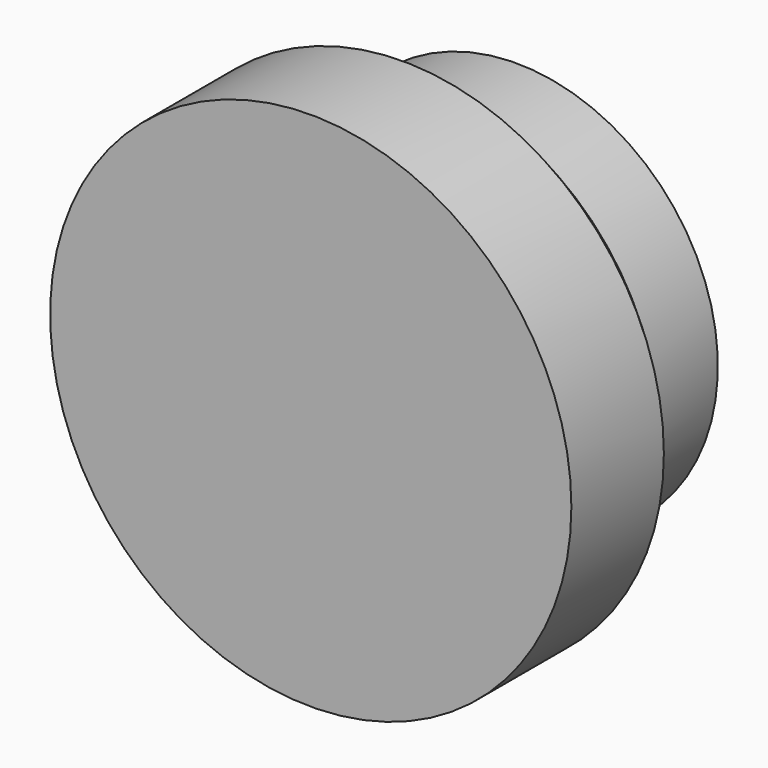
from build123d import *

# Parameters (mm, degrees)
F0_R     = 45.9871931788
F1_DEPTH = 12.7
F4_R     = 35.5142998493
F5_DEPTH = 20
F6_SIZE  = 5


# Not quite as in the source:
# - the program builds the solid bodies; features that only make, move or delete a surface that nothing else refers to are left out


with BuildPart() as f1:
    # F0 (on Front) → F1 (new body, symmetric)
    with BuildSketch(Plane.XZ):
        with Locations((0, 5.3770393133)):
            Circle(F0_R)
    extrude(amount=F1_DEPTH, both=True)

    # F4 (on face) → F5 (join)
    with BuildSketch(Plane(origin=(0, 12.7, 0), x_dir=(-1, 0, 0), z_dir=(0, 1, 0))):
        with Locations((0, 5.3770393133)):
            Circle(F4_R)
    extrude(amount=F5_DEPTH)

    # F6
    f6_edges = [f1.edges().sort_by_distance(p)[0] for p in [
        (-45.987193, 12.7, 5.377039),
    ]]
    chamfer(f6_edges, length=F6_SIZE)


solid = f1.part
